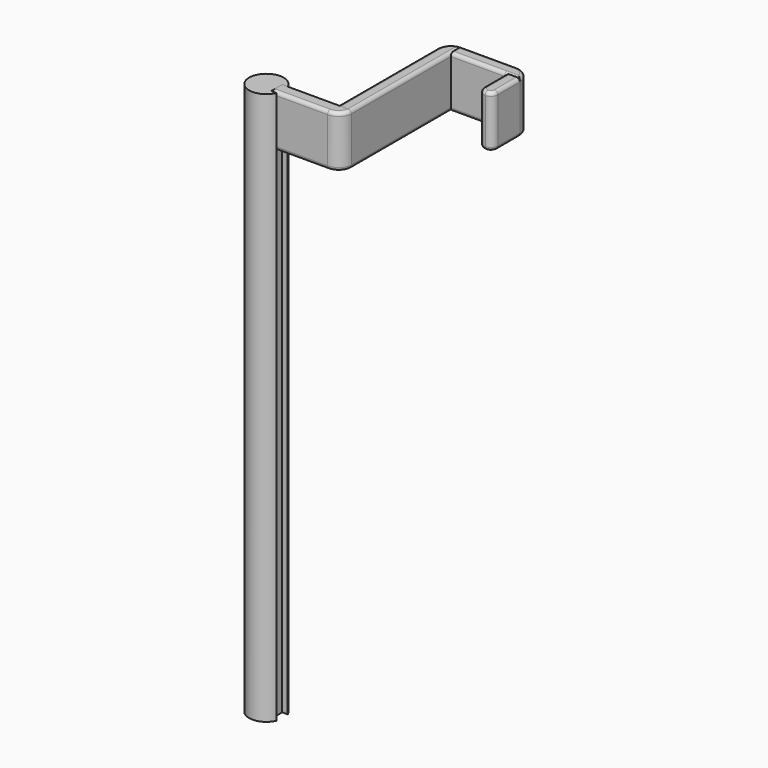
from build123d import *

# Parameters (mm, degrees)
F0_R            = 6.35
F1_DEPTH        = 203.2
F2_W            = 2.54
F2_H            = 2.54
F3_DEPTH        = 227.838
F4_W            = 4.572
F4_H            = 19.05
F5_DEPTH        = 25.4
F6_W            = 5.08
F6_H            = 19.05
F7_DEPTH        = 50.8
F8_W            = 5.08
F8_H            = 19.05
F9_DEPTH        = 25.4
F10_W           = 5.08
F10_H           = 19.05
F11_DEPTH       = 12.7
F12_R           = 5.07999
F12_2_R         = 5.07999
F13_F1_R        = 2.54
F13_F2_R        = 2.5399
F13_2_T1_DEPTH  = 6.3524242923
F13_3_T1_DEPTH  = 6.3524242923
F14_T1_DEPTH    = 44.3226809025
F15_F1_R        = 1.27
F15_F2_R        = 1.27
F15_2_T1_DEPTH  = 54.6541223675
F15_2_T3_DEPTH  = 48.89501
F15_2_T6_ANGLE  = 125.8243178297
F15_2_T8_ANGLE  = 125.8243178297
F15_3_T1_DEPTH  = 8.8507063741
F15_3_T3_DEPTH  = 29.2589511095
F15_3_T5_DEPTH  = 23.4974243709
F15_3_T8_ANGLE  = 125.8515597797
F15_3_T10_ANGLE = 125.8515597797
F15_4_F1_R      = 1.27
F15_4_F2_R      = 1.27


# Not quite as in the source:
# - a fillet or chamfer that OpenCascade refuses, or shapes differently, is made with other operations: its cross-section is extruded or revolved along the edge and cut away or added
# - a fillet or chamfer is up to 0.001 mm smaller than in the source, because OpenCascade refuses the exact size
# - a feature names something its author has since deleted; it is built from what else it names


with BuildPart() as f1:
    # F0 (on Top) → F1 (new body)
    with BuildSketch(Plane.XY):
        with Locations((-37.5121086836, 29.2024631053)):
            Circle(F0_R)
    extrude(amount=F1_DEPTH)

    # F2 (on face) → F3 (cut)
    with BuildSketch(Plane.XY.offset(203.2)):
        with Locations((-32.4321086836, 30.4724631053)):
            Rectangle(F2_W, F2_H)
        with Locations((-32.4321086836, 27.9324631053)):
            Rectangle(F2_W, F2_H)
    extrude(amount=-F3_DEPTH, mode=Mode.SUBTRACT)


with BuildPart() as f5:
    # F4 (on face) → F5 (new body)
    with BuildSketch(Plane.YZ.offset(-33.7021086836)):
        with Locations((29.4564631053, 193.675)):
            Rectangle(F4_W, F4_H)
    extrude(amount=F5_DEPTH)

    # F14: fillet of radius 5.08 on 1 edges, made by hand

    # F14_s2 → F14_t1 (cut)
    with BuildSketch(Plane.XY.offset(171.5136595487)):
        with BuildLine():
            ThreePointArc((-13.3566448641, 27.1704631053), (-9.9488772664, 28.4830342739), (-8.3021086836, 31.7424631053))
            Line((-8.3021086836, 31.7424631053), (-8.3021086836, 27.1704631053))
            Line((-8.3021086836, 27.1704631053), (-13.3566448641, 27.1704631053))
        make_face()
    extrude(amount=F14_T1_DEPTH, mode=Mode.SUBTRACT)

    # F15: fillet of radius 1.27 on 4 edges, made by hand

    # F15_f1
    f15_f1_edges = [f5.edges().sort_by_distance(p)[0] for p in [
        (-9.9488772664, 28.4830342739, 184.15),
        (-23.5293767738, 27.1704631053, 184.15),
    ]]
    fillet(f15_f1_edges, radius=F15_F1_R)

    # F15_f2
    f15_f2_edges = [f5.edges().sort_by_distance(p)[0] for p in [
        (-23.5293767738, 27.1704631053, 203.2),
        (-9.9488772664, 28.4830342739, 203.2),
    ]]
    fillet(f15_f2_edges, radius=F15_F2_R)


with BuildPart() as f7:
    # F6 (on face) → F7 (new body)
    with BuildSketch(Plane(origin=(0, 31.7424631053, 0), x_dir=(-1, 0, 0), z_dir=(0, 1, 0))):
        with Locations((10.8421086836, 193.675)):
            Rectangle(F6_W, F6_H)
    extrude(amount=F7_DEPTH)

    # F12 (radius 5.08 in the source; OpenCascade refuses exactly that, so slightly less here)
    f12_edges = [f7.edges().sort_by_distance(p)[0] for p in [
        (-13.382109, 82.542463, 193.675),
    ]]
    fillet(f12_edges, radius=F12_R)

    # F13#2: fillet of radius 2.54 on 2 edges, made by hand

    # F13_2_s2 → F13_2_t1 (cut)
    with BuildSketch(Plane.YZ.offset(-8.3021186836)):
        with BuildLine():
            ThreePointArc((80.0014974199, 203.2004), (81.7985143295, 202.4560512242), (82.5428631053, 200.6590343146))
            Line((82.5428631053, 200.6590343146), (82.7969996739, 200.6590343146))
            ThreePointArc((82.7969996739, 200.6590343146), (82.7965996739, 201.9295171573), (82.7965996739, 203.2))
            Line((82.7965996739, 203.2), (82.5424631053, 203.4541365685))
            ThreePointArc((82.5424631053, 203.4541365685), (81.2719802626, 203.4541365685), (80.0014974199, 203.4545365685))
            Line((80.0014974199, 203.4545365685), (80.0014974199, 203.2004))
        make_face()
        with BuildLine():
            ThreePointArc((82.5428631053, 186.6909656854), (81.7985143295, 184.8939487758), (80.0014974199, 184.1496))
            Line((80.0014974199, 184.1496), (80.0014974199, 183.8954634315))
            ThreePointArc((80.0014974199, 183.8954634315), (81.2719802626, 183.8958634315), (82.5424631053, 183.8958634315))
            Line((82.5424631053, 183.8958634315), (82.7965996739, 184.15))
            ThreePointArc((82.7965996739, 184.15), (82.7965996739, 185.4204828427), (82.7969996739, 186.6909656854))
            Line((82.7969996739, 186.6909656854), (82.5428631053, 186.6909656854))
        make_face()
    extrude(amount=F13_2_T1_DEPTH, mode=Mode.SUBTRACT)

    # F15#2: fillet of radius 1.27 on 6 edges, made by hand

    # F15_2_s2 → F15_2_t1 (cut)
    with BuildSketch(Plane.XZ.offset(-83.2215854729)):
        with BuildLine():
            ThreePointArc((-9.5721086836, 203.2), (-8.6740830715, 202.8280256121), (-8.3021086836, 201.93))
            Line((-8.3021086836, 201.93), (-8.3021086836, 203.2))
            Line((-8.3021086836, 203.2), (-9.5721086836, 203.2))
        make_face()
        with BuildLine():
            ThreePointArc((-8.3021086836, 185.42), (-8.6740830715, 184.5219743879), (-9.5721086836, 184.15))
            Line((-9.5721086836, 184.15), (-8.3021086836, 184.15))
            Line((-8.3021086836, 184.15), (-8.3021086836, 185.42))
        make_face()
    extrude(amount=F15_2_T1_DEPTH, mode=Mode.SUBTRACT)

    # F15_2_s4 → F15_2_t3 (cut)
    with BuildSketch(Plane.XZ.offset(-77.4624731053)):
        with BuildLine():
            ThreePointArc((-12.1121086836, 203.2), (-13.0101342957, 202.8280256121), (-13.3821086836, 201.93))
            Line((-13.3821086836, 201.93), (-13.3821086836, 203.2))
            Line((-13.3821086836, 203.2), (-12.1121086836, 203.2))
        make_face()
        with BuildLine():
            ThreePointArc((-13.3821086836, 185.42), (-13.0101342957, 184.5219743879), (-12.1121086836, 184.15))
            Line((-12.1121086836, 184.15), (-13.3821086836, 184.15))
            Line((-13.3821086836, 184.15), (-13.3821086836, 185.42))
        make_face()
    extrude(amount=F15_2_T3_DEPTH, mode=Mode.SUBTRACT)

    # F15_2_s5 → F15_2_t6 (revolve, cut)
    with BuildSketch(Plane.XZ.offset(-77.4624731053)):
        with BuildLine():
            ThreePointArc((-13.3821086836, 185.42), (-13.0101342957, 184.5219743879), (-12.1121086836, 184.15))
            Line((-12.1121086836, 184.15), (-13.3821086836, 184.15))
            Line((-13.3821086836, 184.15), (-13.3821086836, 185.42))
        make_face()
    revolve(axis=Axis((-8.3021186836, 77.4624731053, 184.15), (0, 0, -1)), revolution_arc=F15_2_T6_ANGLE, mode=Mode.SUBTRACT)

    # F15_2_s7 → F15_2_t8 (revolve, cut)
    with BuildSketch(Plane.XZ.offset(-77.4624731053)):
        with BuildLine():
            ThreePointArc((-12.1121086836, 203.2), (-13.0101342957, 202.8280256121), (-13.3821086836, 201.93))
            Line((-13.3821086836, 201.93), (-13.3821086836, 203.2))
            Line((-13.3821086836, 203.2), (-12.1121086836, 203.2))
        make_face()
    revolve(axis=Axis((-8.3021186836, 77.4624731053, 203.2), (0, 0, -1)), revolution_arc=F15_2_T8_ANGLE, mode=Mode.SUBTRACT)


with BuildPart() as f9:
    # F8 (on face) → F9 (new body)
    with BuildSketch(Plane.YZ.offset(-8.3021086836)):
        with Locations((80.0024631053, 193.675)):
            Rectangle(F8_W, F8_H)
    extrude(amount=F9_DEPTH)

    # F12#2 (radius 5.08 in the source; OpenCascade refuses exactly that, so slightly less here)
    f12_2_edges = [f9.edges().sort_by_distance(p)[0] for p in [
        (17.097891, 82.542463, 193.675),
    ]]
    fillet(f12_2_edges, radius=F12_2_R)

    # F13#3: fillet of radius 2.54 on 2 edges, made by hand

    # F13_3_s2 → F13_3_t1 (cut)
    with BuildSketch(Plane.XZ.offset(-77.4624731053)):
        with BuildLine():
            ThreePointArc((14.556925631, 184.1496), (16.3539425406, 184.8939487758), (17.0982913164, 186.6909656854))
            Line((17.0982913164, 186.6909656854), (17.352427885, 186.6909656854))
            ThreePointArc((17.352427885, 186.6909656854), (17.352027885, 185.4204828427), (17.352027885, 184.15))
            Line((17.352027885, 184.15), (17.0978913164, 183.8958634315))
            ThreePointArc((17.0978913164, 183.8958634315), (15.8274084737, 183.8958634315), (14.556925631, 183.8954634315))
            Line((14.556925631, 183.8954634315), (14.556925631, 184.1496))
        make_face()
        with BuildLine():
            ThreePointArc((14.556925631, 203.2004), (16.3539425406, 202.4560512242), (17.0982913164, 200.6590343146))
            Line((17.0982913164, 200.6590343146), (17.352427885, 200.6590343146))
            ThreePointArc((17.352427885, 200.6590343146), (17.352027885, 201.9295171573), (17.352027885, 203.2))
            Line((17.352027885, 203.2), (17.0978913164, 203.4541365685))
            ThreePointArc((17.0978913164, 203.4541365685), (15.8274084737, 203.4541365685), (14.556925631, 203.4545365685))
            Line((14.556925631, 203.4545365685), (14.556925631, 203.2004))
        make_face()
    extrude(amount=F13_3_T1_DEPTH, mode=Mode.SUBTRACT)

    # F15#3: fillet of radius 1.27 on 12 edges, made by hand

    # F15_3_s2 → F15_3_t1 (cut)
    with BuildSketch(Plane.YZ.offset(11.4245993133)):
        with BuildLine():
            ThreePointArc((78.7334387907, 203.2004), (77.8344474932, 202.8280256121), (77.4620731053, 201.9290343146))
            Line((77.4620731053, 201.9290343146), (77.3349365368, 201.9290343146))
            ThreePointArc((77.3349365368, 201.9290343146), (77.3353365368, 202.5645171573), (77.3353365368, 203.2))
            Line((77.3353365368, 203.2), (77.4624731053, 203.3271365685))
            ThreePointArc((77.4624731053, 203.3271365685), (78.097955948, 203.3271365685), (78.7334387907, 203.3275365685))
            Line((78.7334387907, 203.3275365685), (78.7334387907, 203.2004))
        make_face()
        with BuildLine():
            ThreePointArc((78.7334387907, 184.1496), (77.8344474932, 184.5219743879), (77.4620731053, 185.4209656854))
            Line((77.4620731053, 185.4209656854), (77.3349365368, 185.4209656854))
            ThreePointArc((77.3349365368, 185.4209656854), (77.3353365368, 184.7854828427), (77.3353365368, 184.15))
            Line((77.3353365368, 184.15), (77.4624731053, 184.0228634315))
            ThreePointArc((77.4624731053, 184.0228634315), (78.097955948, 184.0228634315), (78.7334387907, 184.0224634315))
            Line((78.7334387907, 184.0224634315), (78.7334387907, 184.1496))
        make_face()
    extrude(amount=F15_3_T1_DEPTH, mode=Mode.SUBTRACT)

    # F15_3_s4 → F15_3_t3 (cut)
    with BuildSketch(Plane.YZ.offset(-11.4795230545)):
        with BuildLine():
            ThreePointArc((78.7334287907, 203.2004), (77.8344374932, 202.8280256121), (77.4620631053, 201.9290343146))
            Line((77.4620631053, 201.9290343146), (77.3349265368, 201.9290343146))
            ThreePointArc((77.3349265368, 201.9290343146), (77.3353265368, 202.5645171573), (77.3353265368, 203.2))
            Line((77.3353265368, 203.2), (77.4624631053, 203.3271365685))
            ThreePointArc((77.4624631053, 203.3271365685), (78.097945948, 203.3271365685), (78.7334287907, 203.3275365685))
            Line((78.7334287907, 203.3275365685), (78.7334287907, 203.2004))
        make_face()
        with BuildLine():
            ThreePointArc((78.7334287907, 184.1496), (77.8344374932, 184.5219743879), (77.4620631053, 185.4209656854))
            Line((77.4620631053, 185.4209656854), (77.3349265368, 185.4209656854))
            ThreePointArc((77.3349265368, 185.4209656854), (77.3353265368, 184.7854828427), (77.3353265368, 184.15))
            Line((77.3353265368, 184.15), (77.4624631053, 184.0228634315))
            ThreePointArc((77.4624631053, 184.0228634315), (78.097945948, 184.0228634315), (78.7334287907, 184.0224634315))
            Line((78.7334287907, 184.0224634315), (78.7334287907, 184.1496))
        make_face()
    extrude(amount=F15_3_T3_DEPTH, mode=Mode.SUBTRACT)

    # F15_3_s6 → F15_3_t5 (cut)
    with BuildSketch(Plane.YZ.offset(-11.4795230545)):
        with BuildLine():
            ThreePointArc((82.5428631053, 201.9290343146), (82.1704887174, 202.8280256121), (81.2714974199, 203.2004))
            Line((81.2714974199, 203.2004), (81.2714974199, 203.3275365685))
            ThreePointArc((81.2714974199, 203.3275365685), (81.9069802626, 203.3271365685), (82.5424631053, 203.3271365685))
            Line((82.5424631053, 203.3271365685), (82.6695996739, 203.2))
            ThreePointArc((82.6695996739, 203.2), (82.6695996739, 202.5645171573), (82.6699996739, 201.9290343146))
            Line((82.6699996739, 201.9290343146), (82.5428631053, 201.9290343146))
        make_face()
        with BuildLine():
            ThreePointArc((82.5428631053, 185.4209656854), (82.1704887174, 184.5219743879), (81.2714974199, 184.1496))
            Line((81.2714974199, 184.1496), (81.2714974199, 184.0224634315))
            ThreePointArc((81.2714974199, 184.0224634315), (81.9069802626, 184.0228634315), (82.5424631053, 184.0228634315))
            Line((82.5424631053, 184.0228634315), (82.6695996739, 184.15))
            ThreePointArc((82.6695996739, 184.15), (82.6695996739, 184.7854828427), (82.6699996739, 185.4209656854))
            Line((82.6699996739, 185.4209656854), (82.5428631053, 185.4209656854))
        make_face()
    extrude(amount=F15_3_T5_DEPTH, mode=Mode.SUBTRACT)

    # F15_3_s7 → F15_3_t8 (revolve, cut)
    with BuildSketch(Plane.YZ.offset(12.0179013164)):
        with BuildLine():
            ThreePointArc((81.2714974199, 184.1496), (82.1704887174, 184.5219743879), (82.5428631053, 185.4209656854))
            Line((82.5428631053, 185.4209656854), (82.6699996739, 185.4209656854))
            ThreePointArc((82.6699996739, 185.4209656854), (82.6695996739, 184.7854828427), (82.6695996739, 184.15))
            Line((82.6695996739, 184.15), (82.5424631053, 184.0228634315))
            ThreePointArc((82.5424631053, 184.0228634315), (81.9069802626, 184.0228634315), (81.2714974199, 184.0224634315))
            Line((81.2714974199, 184.0224634315), (81.2714974199, 184.1496))
        make_face()
    revolve(axis=Axis((12.0179013164, 77.4624731053, 184.15), (0, 0, -1)), revolution_arc=F15_3_T8_ANGLE, mode=Mode.SUBTRACT)

    # F15_3_s9 → F15_3_t10 (revolve, cut)
    with BuildSketch(Plane.YZ.offset(12.0179013164)):
        with BuildLine():
            ThreePointArc((82.5428631053, 201.9290343146), (82.1704887174, 202.8280256121), (81.2714974199, 203.2004))
            Line((81.2714974199, 203.2004), (81.2714974199, 203.3275365685))
            ThreePointArc((81.2714974199, 203.3275365685), (81.9069802626, 203.3271365685), (82.5424631053, 203.3271365685))
            Line((82.5424631053, 203.3271365685), (82.6695996739, 203.2))
            ThreePointArc((82.6695996739, 203.2), (82.6695996739, 202.5645171573), (82.6699996739, 201.9290343146))
            Line((82.6699996739, 201.9290343146), (82.5428631053, 201.9290343146))
        make_face()
    revolve(axis=Axis((12.0179013164, 77.4624731053, 203.2), (0, 0, -1)), revolution_arc=F15_3_T10_ANGLE, mode=Mode.SUBTRACT)


with BuildPart() as f11:
    # F10 (on face) → F11 (new body)
    with BuildSketch(Plane.XZ.offset(-77.4624631053)):
        with Locations((14.5578913164, 193.675)):
            Rectangle(F10_W, F10_H)
    extrude(amount=F11_DEPTH)

    # F13: fillet of radius 2.54 on 2 edges, made by hand

    # F13_f1
    f13_f1_edges = [f11.edges().sort_by_distance(p)[0] for p in [
        (17.0978913164, 64.7624631053, 193.675),
    ]]
    fillet(f13_f1_edges, radius=F13_F1_R)

    # F13_f2 (radius 2.54 in the source; OpenCascade refuses exactly that, so slightly less here)
    f13_f2_edges = [f11.edges().sort_by_distance(p)[0] for p in [
        (12.0178913164, 64.7624631053, 193.675),
    ]]
    fillet(f13_f2_edges, radius=F13_F2_R)

    # F15#4: fillet of radius 1.27 on 10 edges, made by hand

    # F15_4_f1
    f15_4_f1_edges = [f11.edges().sort_by_distance(p)[0] for p in [
        (14.5578413164, 64.7624631053, 184.15),
        (12.7618108029, 65.5063825918, 184.15),
        (16.3539425406, 65.5064118811, 184.15),
        (12.0178913164, 72.3824131053, 184.15),
        (17.0978913164, 72.3824631053, 184.15),
    ]]
    fillet(f15_4_f1_edges, radius=F15_4_F1_R)

    # F15_4_f2
    f15_4_f2_edges = [f11.edges().sort_by_distance(p)[0] for p in [
        (14.5578413164, 64.7624631053, 203.2),
        (12.7618108029, 65.5063825918, 203.2),
        (16.3539425406, 65.5064118811, 203.2),
        (12.0178913164, 72.3824131053, 203.2),
        (17.0978913164, 72.3824631053, 203.2),
    ]]
    fillet(f15_4_f2_edges, radius=F15_4_F2_R)


solid = Compound([f1.part, f5.part, f7.part, f9.part, f11.part])
